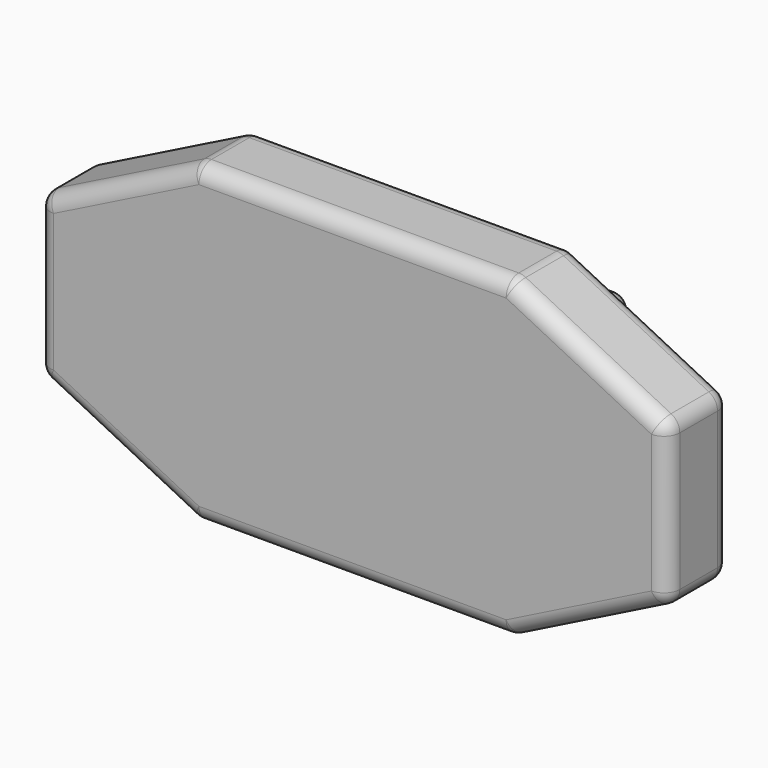
from build123d import *

# Parameters (mm, degrees)
F1_DEPTH     = 25.4
F2_R         = 5.08
F3_R         = 5.08
F4_W         = 12.7
F4_H         = 50.8
F5_DEPTH     = 25.4
F6_W         = 18.1257220684
F6_H         = 38.8130061328
F7_DEPTH     = 254
F8_T1_DEPTH  = 2.54
F8_T3_DEPTH  = 40.64
F8_T5_DEPTH  = 20.32
F8_S9_W      = 5.08
F8_S9_H      = 5.08
F8_T10_DEPTH = 5.08
F8_S15_W     = 5.08
F8_S15_H     = 5.08
F8_T16_DEPTH = 5.08
F8_S21_W     = 5.08
F8_S21_H     = 5.08
F8_T22_DEPTH = 5.08
F8_S27_W     = 5.08
F8_S27_H     = 5.08
F8_T28_DEPTH = 5.08
F9_T1_DEPTH  = 40.64
F9_T3_DEPTH  = 2.54
F9_T5_DEPTH  = 20.32
F9_S9_W      = 5.08
F9_S9_H      = 5.08
F9_T10_DEPTH = 5.08
F9_S15_W     = 5.08
F9_S15_H     = 5.08
F9_T16_DEPTH = 5.08
F9_S21_W     = 5.08
F9_S21_H     = 5.08
F9_T22_DEPTH = 5.08
F9_S27_W     = 5.08
F9_S27_H     = 5.08
F9_T28_DEPTH = 5.08


# Not quite as in the source:
# - a fillet or chamfer that OpenCascade refuses, or shapes differently, is made with other operations: its cross-section is extruded or revolved along the edge and cut away or added


with BuildPart() as f1:
    # F0 (on Front) → F1 (new body)
    with BuildSketch(Plane.XZ):
        Polygon((-101.6, -25.4), (-50.8, -50.8), (50.8, -50.8), (101.6, -25.4), (101.6, 25.4), (50.8, 50.8), (-50.8, 50.8), (-101.6, 25.4), align=None)
    extrude(amount=F1_DEPTH)

    # F2
    f2_edges = [f1.edges().sort_by_distance(p)[0] for p in [
        (-76.2, -25.4, 38.1),
        (0, -25.4, 50.8),
        (76.2, -25.4, 38.1),
        (101.6, -25.4, 0),
        (-76.2, -25.4, -38.1),
        (0, -25.4, -50.8),
        (76.2, -25.4, -38.1),
        (-101.6, -25.4, 0),
        (-50.8, -12.7, -50.8),
        (-101.6, -12.7, -25.4),
        (-101.6, -12.7, 25.4),
        (-50.8, -12.7, 50.8),
        (50.8, -12.7, 50.8),
        (101.6, -12.7, 25.4),
        (101.6, -12.7, -25.4),
        (50.8, -12.7, -50.8),
    ]]
    fillet(f2_edges, radius=F2_R)

    # F3
    f3_edges = [f1.edges().sort_by_distance(p)[0] for p in [
        (-75.332232, 0, -38.533884),
        (-100.841306, 0, -24.931101),
        (-50.76792, 0, -50.664105),
        (-101.6, 0, 0),
        (0, 0, -50.8),
        (-100.841306, 0, 24.931101),
        (50.76792, 0, -50.664105),
        (-75.332232, 0, 38.533884),
        (75.332232, 0, -38.533884),
        (-50.76792, 0, 50.664105),
        (100.841306, 0, -24.931101),
        (0, 0, 50.8),
        (101.6, 0, 0),
        (50.76792, 0, 50.664105),
        (100.841306, 0, 24.931101),
        (75.332232, 0, 38.533884),
    ]]
    fillet(f3_edges, radius=F3_R)

    # F4 (on face) → F5 (join)
    with BuildSketch(Plane(origin=(0, 0, 0), x_dir=(-1, 0, 0), z_dir=(0, 1, 0))):
        with Locations((-43.9901705831, 1.8079679169)):
            Rectangle(F4_W, F4_H)
        with Locations((43.9901705831, 1.8079679169)):
            Rectangle(F4_W, F4_H)
    extrude(amount=F5_DEPTH)

    # F6 (on face) → F7 (cut)
    with BuildSketch(Plane(origin=(-50.3401705831, 0, 0), x_dir=(0, -1, 0), z_dir=(-1, 0, 0))):
        with Locations((-10.3619872243, 2.8695575893)):
            Rectangle(F6_W, F6_H)
    extrude(amount=-F7_DEPTH, mode=Mode.SUBTRACT)

    # F8: fillet of radius 5.08 on 8 edges, made by hand

    # F8_s2 → F8_t1 (cut)
    with BuildSketch(Plane.YZ.offset(42.7201705831)):
        with BuildLine():
            ThreePointArc((20.32, 27.2079679169), (23.9121024484, 25.7200703653), (25.4, 22.1279679169))
            Line((25.4, 22.1279679169), (25.4, 27.2079679169))
            Line((25.4, 27.2079679169), (20.32, 27.2079679169))
        make_face()
        with BuildLine():
            ThreePointArc((20.32, -23.5920320831), (23.9121024484, -22.1041345315), (25.4, -18.5120320831))
            Line((25.4, -18.5120320831), (25.4, -23.5920320831))
            Line((25.4, -23.5920320831), (20.32, -23.5920320831))
        make_face()
    extrude(amount=F8_T1_DEPTH, mode=Mode.SUBTRACT)

    # F8_s4 → F8_t3 (cut)
    with BuildSketch(Plane.XY.offset(-18.5120320831)):
        with BuildLine():
            ThreePointArc((50.3401705831, 20.32), (48.8522730316, 23.9121024484), (45.2601705831, 25.4))
            Line((45.2601705831, 25.4), (50.3401705831, 25.4))
            Line((50.3401705831, 25.4), (50.3401705831, 20.32))
        make_face()
        with BuildLine():
            ThreePointArc((37.6401705831, 20.32), (39.1280681347, 23.9121024484), (42.7201705831, 25.4))
            Line((42.7201705831, 25.4), (37.6401705831, 25.4))
            Line((37.6401705831, 25.4), (37.6401705831, 20.32))
        make_face()
    extrude(amount=F8_T3_DEPTH, mode=Mode.SUBTRACT)

    # F8_s6 → F8_t5 (cut)
    with BuildSketch(Plane.XZ.offset(-20.32)):
        with BuildLine():
            ThreePointArc((45.2601705831, -23.5920320831), (48.8522730316, -22.1041345315), (50.3401705831, -18.5120320831))
            Line((50.3401705831, -18.5120320831), (50.3401705831, -23.5920320831))
            Line((50.3401705831, -23.5920320831), (45.2601705831, -23.5920320831))
        make_face()
        with BuildLine():
            ThreePointArc((37.6401705831, -18.5120320831), (39.1280681347, -22.1041345315), (42.7201705831, -23.5920320831))
            Line((42.7201705831, -23.5920320831), (37.6401705831, -23.5920320831))
            Line((37.6401705831, -23.5920320831), (37.6401705831, -18.5120320831))
        make_face()
        with BuildLine():
            ThreePointArc((37.6401705831, 22.1279679169), (39.1280681347, 25.7200703653), (42.7201705831, 27.2079679169))
            Line((42.7201705831, 27.2079679169), (37.6401705831, 27.2079679169))
            Line((37.6401705831, 27.2079679169), (37.6401705831, 22.1279679169))
        make_face()
        with BuildLine():
            ThreePointArc((50.3401705831, 22.1279679169), (48.8522730316, 25.7200703653), (45.2601705831, 27.2079679169))
            Line((45.2601705831, 27.2079679169), (50.3401705831, 27.2079679169))
            Line((50.3401705831, 27.2079679169), (50.3401705831, 22.1279679169))
        make_face()
    extrude(amount=F8_T5_DEPTH, mode=Mode.SUBTRACT)


with BuildPart() as f8_tool8:
    # F8_s9 → F8_t10 (new body)
    with BuildSketch(Plane.YZ.offset(42.7201705831)):
        with Locations((22.86, 24.6679679169)):
            Rectangle(F8_S9_W, F8_S9_H)
    extrude(amount=-F8_T10_DEPTH)

    # F8_s11 → F8_t12 (revolve, cut)
    with BuildSketch(Plane(origin=(42.7201705831, 20.32, 22.1279679169), x_dir=(0, -0.7071067812, -0.7071067812), z_dir=(0, 0.7071067812, -0.7071067812))):
        with BuildLine():
            ThreePointArc((0, -5.08), (5.08, 0), (0, 5.08))
            Line((0, 5.08), (0, -5.08))
        make_face()
    revolve(axis=Axis((42.7201705831, 20.32, 22.1279679169), (-1, 0, 0)), mode=Mode.SUBTRACT)


with BuildPart() as f1_1:
    add(f1.part)

    # F8_t7: cut F8_tool8
    add(f8_tool8.part, mode=Mode.SUBTRACT)


with BuildPart() as f8_tool14:
    # F8_s15 → F8_t16 (new body)
    with BuildSketch(Plane.YZ.offset(45.2601705831)):
        with Locations((22.86, 24.6679679169)):
            Rectangle(F8_S15_W, F8_S15_H)
    extrude(amount=F8_T16_DEPTH)

    # F8_s17 → F8_t18 (revolve, cut)
    with BuildSketch(Plane(origin=(45.2601705831, 20.32, 22.1279679169), x_dir=(0, -0.7071067812, -0.7071067812), z_dir=(0, -0.7071067812, 0.7071067812))):
        with BuildLine():
            ThreePointArc((0, -5.08), (5.08, 0), (0, 5.08))
            Line((0, 5.08), (0, -5.08))
        make_face()
    revolve(axis=Axis((45.2601705831, 20.32, 22.1279679169), (1, 0, 0)), mode=Mode.SUBTRACT)


with BuildPart() as f1_2:
    add(f1_1.part)

    # F8_t13: cut F8_tool14
    add(f8_tool14.part, mode=Mode.SUBTRACT)


with BuildPart() as f8_tool20:
    # F8_s21 → F8_t22 (new body)
    with BuildSketch(Plane.XY.offset(-18.5120320831)):
        with Locations((47.8001705831, 22.86)):
            Rectangle(F8_S21_W, F8_S21_H)
    extrude(amount=-F8_T22_DEPTH)

    # F8_s23 → F8_t24 (revolve, cut)
    with BuildSketch(Plane(origin=(45.2601705831, 20.32, -18.5120320831), x_dir=(-0.7071067812, -0.7071067812, 0), z_dir=(0.7071067812, -0.7071067812, 0))):
        with BuildLine():
            ThreePointArc((0, -5.08), (5.08, 0), (0, 5.08))
            Line((0, 5.08), (0, -5.08))
        make_face()
    revolve(axis=Axis((45.2601705831, 20.32, -18.5120320831), (0, 0, -1)), mode=Mode.SUBTRACT)


with BuildPart() as f1_3:
    add(f1_2.part)

    # F8_t19: cut F8_tool20
    add(f8_tool20.part, mode=Mode.SUBTRACT)


with BuildPart() as f8_tool26:
    # F8_s27 → F8_t28 (new body)
    with BuildSketch(Plane.YZ.offset(42.7201705831)):
        with Locations((22.86, -21.0520320831)):
            Rectangle(F8_S27_W, F8_S27_H)
    extrude(amount=-F8_T28_DEPTH)

    # F8_s29 → F8_t30 (revolve, cut)
    with BuildSketch(Plane(origin=(42.7201705831, 20.32, -18.5120320831), x_dir=(0, -0.7071067812, 0.7071067812), z_dir=(0, -0.7071067812, -0.7071067812))):
        with BuildLine():
            ThreePointArc((0, -5.08), (5.08, 0), (0, 5.08))
            Line((0, 5.08), (0, -5.08))
        make_face()
    revolve(axis=Axis((42.7201705831, 20.32, -18.5120320831), (-1, 0, 0)), mode=Mode.SUBTRACT)


with BuildPart() as f1_4:
    add(f1_3.part)

    # F8_t25: cut F8_tool26
    add(f8_tool26.part, mode=Mode.SUBTRACT)

    # F9: fillet of radius 5.08 on 8 edges, made by hand

    # F9_s2 → F9_t1 (cut)
    with BuildSketch(Plane.XY.offset(-18.5120320831)):
        with BuildLine():
            ThreePointArc((-37.6401705831, 20.32), (-39.1280681347, 23.9121024484), (-42.7201705831, 25.4))
            Line((-42.7201705831, 25.4), (-37.6401705831, 25.4))
            Line((-37.6401705831, 25.4), (-37.6401705831, 20.32))
        make_face()
        with BuildLine():
            ThreePointArc((-50.3401705831, 20.32), (-48.8522730316, 23.9121024484), (-45.2601705831, 25.4))
            Line((-45.2601705831, 25.4), (-50.3401705831, 25.4))
            Line((-50.3401705831, 25.4), (-50.3401705831, 20.32))
        make_face()
    extrude(amount=F9_T1_DEPTH, mode=Mode.SUBTRACT)

    # F9_s4 → F9_t3 (cut)
    with BuildSketch(Plane.YZ.offset(-45.2601705831)):
        with BuildLine():
            ThreePointArc((20.32, -23.5920320831), (23.9121024484, -22.1041345315), (25.4, -18.5120320831))
            Line((25.4, -18.5120320831), (25.4, -23.5920320831))
            Line((25.4, -23.5920320831), (20.32, -23.5920320831))
        make_face()
        with BuildLine():
            ThreePointArc((20.32, 27.2079679169), (23.9121024484, 25.7200703653), (25.4, 22.1279679169))
            Line((25.4, 22.1279679169), (25.4, 27.2079679169))
            Line((25.4, 27.2079679169), (20.32, 27.2079679169))
        make_face()
    extrude(amount=F9_T3_DEPTH, mode=Mode.SUBTRACT)

    # F9_s6 → F9_t5 (cut)
    with BuildSketch(Plane.XZ.offset(-20.32)):
        with BuildLine():
            ThreePointArc((-37.6401705831, -18.5120320831), (-39.1280681347, -22.1041345315), (-42.7201705831, -23.5920320831))
            Line((-42.7201705831, -23.5920320831), (-37.6401705831, -23.5920320831))
            Line((-37.6401705831, -23.5920320831), (-37.6401705831, -18.5120320831))
        make_face()
        with BuildLine():
            ThreePointArc((-45.2601705831, -23.5920320831), (-48.8522730316, -22.1041345315), (-50.3401705831, -18.5120320831))
            Line((-50.3401705831, -18.5120320831), (-50.3401705831, -23.5920320831))
            Line((-50.3401705831, -23.5920320831), (-45.2601705831, -23.5920320831))
        make_face()
        with BuildLine():
            ThreePointArc((-42.7201705831, 27.2079679169), (-39.1280681347, 25.7200703653), (-37.6401705831, 22.1279679169))
            Line((-37.6401705831, 22.1279679169), (-37.6401705831, 27.2079679169))
            Line((-37.6401705831, 27.2079679169), (-42.7201705831, 27.2079679169))
        make_face()
        with BuildLine():
            ThreePointArc((-45.2601705831, 27.2079679169), (-48.8522730316, 25.7200703653), (-50.3401705831, 22.1279679169))
            Line((-50.3401705831, 22.1279679169), (-50.3401705831, 27.2079679169))
            Line((-50.3401705831, 27.2079679169), (-45.2601705831, 27.2079679169))
        make_face()
    extrude(amount=F9_T5_DEPTH, mode=Mode.SUBTRACT)


with BuildPart() as f9_tool8:
    # F9_s9 → F9_t10 (new body)
    with BuildSketch(Plane.XZ.offset(-20.32)):
        with Locations((-40.1801705831, 24.6679679169)):
            Rectangle(F9_S9_W, F9_S9_H)
    extrude(amount=-F9_T10_DEPTH)

    # F9_s11 → F9_t12 (revolve, cut)
    with BuildSketch(Plane(origin=(-42.7201705831, 20.32, 22.1279679169), x_dir=(-0.7071067812, 0, -0.7071067812), z_dir=(0.7071067812, 0, -0.7071067812))):
        with BuildLine():
            ThreePointArc((0, -5.08), (5.08, 0), (0, 5.08))
            Line((0, 5.08), (0, -5.08))
        make_face()
    revolve(axis=Axis((-42.7201705831, 20.32, 22.1279679169), (0, 1, 0)), mode=Mode.SUBTRACT)


with BuildPart() as f1_5:
    add(f1_4.part)

    # F9_t7: cut F9_tool8
    add(f9_tool8.part, mode=Mode.SUBTRACT)


with BuildPart() as f9_tool14:
    # F9_s15 → F9_t16 (new body)
    with BuildSketch(Plane.XY.offset(-18.5120320831)):
        with Locations((-40.1801705831, 22.86)):
            Rectangle(F9_S15_W, F9_S15_H)
    extrude(amount=-F9_T16_DEPTH)

    # F9_s17 → F9_t18 (revolve, cut)
    with BuildSketch(Plane(origin=(-42.7201705831, 20.32, -18.5120320831), x_dir=(-0.7071067812, -0.7071067812, 0), z_dir=(0.7071067812, -0.7071067812, 0))):
        with BuildLine():
            ThreePointArc((0, -5.08), (5.08, 0), (0, 5.08))
            Line((0, 5.08), (0, -5.08))
        make_face()
    revolve(axis=Axis((-42.7201705831, 20.32, -18.5120320831), (0, 0, -1)), mode=Mode.SUBTRACT)


with BuildPart() as f1_6:
    add(f1_5.part)

    # F9_t13: cut F9_tool14
    add(f9_tool14.part, mode=Mode.SUBTRACT)


with BuildPart() as f9_tool20:
    # F9_s21 → F9_t22 (new body)
    with BuildSketch(Plane.XY.offset(-18.5120320831)):
        with Locations((-47.8001705831, 22.86)):
            Rectangle(F9_S21_W, F9_S21_H)
    extrude(amount=-F9_T22_DEPTH)

    # F9_s23 → F9_t24 (revolve, cut)
    with BuildSketch(Plane(origin=(-45.2601705831, 20.32, -18.5120320831), x_dir=(0.7071067812, -0.7071067812, 0), z_dir=(0.7071067812, 0.7071067812, 0))):
        with BuildLine():
            ThreePointArc((0, -5.08), (5.08, 0), (0, 5.08))
            Line((0, 5.08), (0, -5.08))
        make_face()
    revolve(axis=Axis((-45.2601705831, 20.32, -18.5120320831), (0, 0, -1)), mode=Mode.SUBTRACT)


with BuildPart() as f1_7:
    add(f1_6.part)

    # F9_t19: cut F9_tool20
    add(f9_tool20.part, mode=Mode.SUBTRACT)


with BuildPart() as f9_tool26:
    # F9_s27 → F9_t28 (new body)
    with BuildSketch(Plane.YZ.offset(-45.2601705831)):
        with Locations((22.86, 24.6679679169)):
            Rectangle(F9_S27_W, F9_S27_H)
    extrude(amount=-F9_T28_DEPTH)

    # F9_s29 → F9_t30 (revolve, cut)
    with BuildSketch(Plane(origin=(-45.2601705831, 20.32, 22.1279679169), x_dir=(0, -0.7071067812, -0.7071067812), z_dir=(0, 0.7071067812, -0.7071067812))):
        with BuildLine():
            ThreePointArc((0, -5.08), (5.08, 0), (0, 5.08))
            Line((0, 5.08), (0, -5.08))
        make_face()
    revolve(axis=Axis((-45.2601705831, 20.32, 22.1279679169), (-1, 0, 0)), mode=Mode.SUBTRACT)


with BuildPart() as f1_8:
    add(f1_7.part)

    # F9_t25: cut F9_tool26
    add(f9_tool26.part, mode=Mode.SUBTRACT)


solid = f1_8.part
